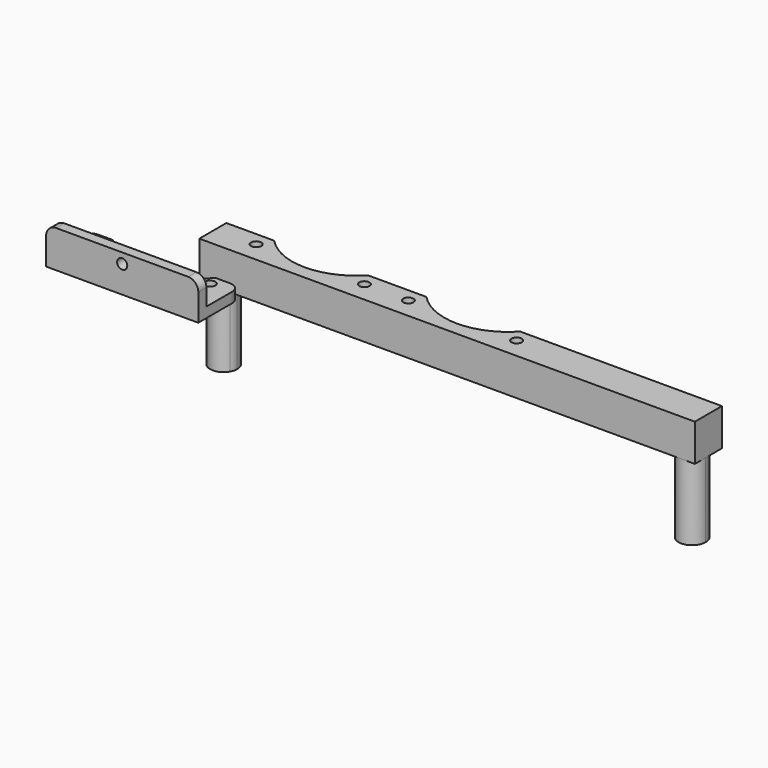
from build123d import *

# Parameters (mm, degrees)
F0_R      = 1.5
F1_DEPTH  = 3
F3_DEPTH  = 8
F5_DEPTH  = 30
F6_R      = 1.5
F7_DEPTH  = 10
F8_W      = 45
F8_H      = 45
F8_R      = 1.55
F8_R_2    = 20
F9_DEPTH  = 3
F10_W     = 45
F10_H     = 6
F11_DEPTH = 3
F12_W     = 45
F12_H     = 3
F13_DEPTH = 8
F14_R     = 1.5
F15_DEPTH = 3.001
F16_R     = 1.55
F17_DEPTH = 33.001
F18_R     = 3


with BuildPart() as f1:
    # F0 (on Top) → F1 (new body)
    with BuildSketch(Plane.XY):
        with BuildLine():
            Line((0, 10), (0, 0))
            Line((0, 0), (146.5, 0))
            Line((146.5, 0), (146.5, 10))
            Line((146.5, 10), (86.8564064606, 10))
            ThreePointArc((86.8564064606, 10), (73, 4), (59.1435935394, 10))
            Line((59.1435935394, 10), (41.8564064606, 10))
            ThreePointArc((41.8564064606, 10), (28, 4), (14.1435935394, 10))
            Line((14.1435935394, 10), (0, 10))
        make_face()
        with Locations((12, 6)):
            Circle(F0_R, mode=Mode.SUBTRACT)
        with Locations((44, 6)):
            Circle(F0_R, mode=Mode.SUBTRACT)
        with Locations((57, 6)):
            Circle(F0_R, mode=Mode.SUBTRACT)
        with Locations((89, 6)):
            Circle(F0_R, mode=Mode.SUBTRACT)
    extrude(amount=F1_DEPTH)

    # F2 (on face) → F3 (join)
    with BuildSketch(Plane(origin=(0, 0, 0), x_dir=(1, 0, 0), z_dir=(0, 0, -1))):
        Polygon((146.5, 0), (0, 0), (0, -10), (2, -10), (2, -2), (144.5, -2), (144.5, -10), (146.5, -10), align=None)
    extrude(amount=F3_DEPTH)

    # F4 (on face) → F5 (join)
    with BuildSketch(Plane(origin=(0, 0, 0), x_dir=(1, 0, 0), z_dir=(0, 0, -1))):
        with BuildLine():
            ThreePointArc((8, -4), (7.8637033052, -2.9647238196), (7.4641016151, -2))
            Line((7.4641016151, -2), (2, -2))
            Line((2, -2), (2, -7.4641016151))
            ThreePointArc((2, -7.4641016151), (6, -7.4641016151), (8, -4))
        make_face()
        with BuildLine():
            Line((144.5, -2), (139.0358983849, -2))
            ThreePointArc((139.0358983849, -2), (139.6715728753, -6.8284271247), (144.5, -7.4641016151))
            Line((144.5, -7.4641016151), (144.5, -2))
        make_face()
        with BuildLine():
            Line((2, -2), (7.4641016151, -2))
            ThreePointArc((7.4641016151, -2), (1.1715728753, -1.1715728753), (2, -7.4641016151))
            Line((2, -7.4641016151), (2, -2))
        make_face()
        with BuildLine():
            ThreePointArc((144.5, -7.4641016151), (145.9641016151, -6), (146.5, -4))
            ThreePointArc((146.5, -4), (143.5352761804, -0.1362966948), (139.0358983849, -2))
            Line((139.0358983849, -2), (144.5, -2))
            Line((144.5, -2), (144.5, -7.4641016151))
        make_face()
    extrude(amount=F5_DEPTH)

    # F6 (on face) → F7 (cut)
    with BuildSketch(Plane(origin=(0, 0, -30), x_dir=(1, 0, 0), z_dir=(0, 0, -1))):
        with Locations((142.5, -4)):
            Circle(F6_R)
        with Locations((4, -4)):
            Circle(F6_R)
    extrude(amount=-F7_DEPTH, mode=Mode.SUBTRACT)


with BuildPart() as f9:
    # F8 (on Top) → F9 (new body)
    with BuildSketch(Plane.XY):
        Rectangle(F8_W, F8_H)
        with Locations((-16, -16)):
            Circle(F8_R, mode=Mode.SUBTRACT)
        with Locations((16, -16)):
            Circle(F8_R, mode=Mode.SUBTRACT)
        with Locations((-16, 16)):
            Circle(F8_R, mode=Mode.SUBTRACT)
        Circle(F8_R_2, mode=Mode.SUBTRACT)
        with Locations((16, 16)):
            Circle(F8_R, mode=Mode.SUBTRACT)
    extrude(amount=F9_DEPTH)

    # F10 (on Top) → F11 (join, through all)
    with BuildSketch(Plane.XY):
        with Locations((0, -25.5)):
            Rectangle(F10_W, F10_H)
    extrude(amount=F11_DEPTH)

    # F12 (on face) → F13 (join)
    with BuildSketch(Plane.XY.offset(3)):
        with Locations((0, -27)):
            Rectangle(F12_W, F12_H)
    extrude(amount=F13_DEPTH)

    # F14 (on face) → F15 (cut, through all)
    with BuildSketch(Plane(origin=(0, -25.5, 0), x_dir=(-1, 0, 0), z_dir=(0, 1, 0))):
        with Locations((0, 8)):
            Circle(F14_R)
    extrude(amount=-F15_DEPTH, mode=Mode.SUBTRACT)

    # F16 (on face) → F17 (cut, through all)
    with BuildSketch(Plane.XY.offset(3)):
        with BuildLine():
            Line((-22.5, 22.5), (-22.5, -13))
            Line((-22.5, -13), (-15.1986841536, -13))
            ThreePointArc((-15.1986841536, -13), (-6.9291527956, 18.7613123618), (20, 0))
            ThreePointArc((20, 0), (18.7613123618, -6.9291527956), (15.1986841536, -13))
            Line((15.1986841536, -13), (22.5, -13))
            Line((22.5, -13), (22.5, 22.5))
            Line((22.5, 22.5), (-22.5, 22.5))
        make_face()
        with Locations((-16, 16)):
            Circle(F16_R, mode=Mode.SUBTRACT)
        with Locations((16, 16)):
            Circle(F16_R, mode=Mode.SUBTRACT)
    extrude(amount=-F17_DEPTH, mode=Mode.SUBTRACT)

    # F18
    f18_edges = [f9.edges().sort_by_distance(p)[0] for p in [
        (22.5, -13, 1.5),
        (-22.5, -13, 1.5),
        (22.5, -27, 11),
        (-22.5, -27, 11),
    ]]
    fillet(f18_edges, radius=F18_R)


solid = Compound([f1.part, f9.part])
